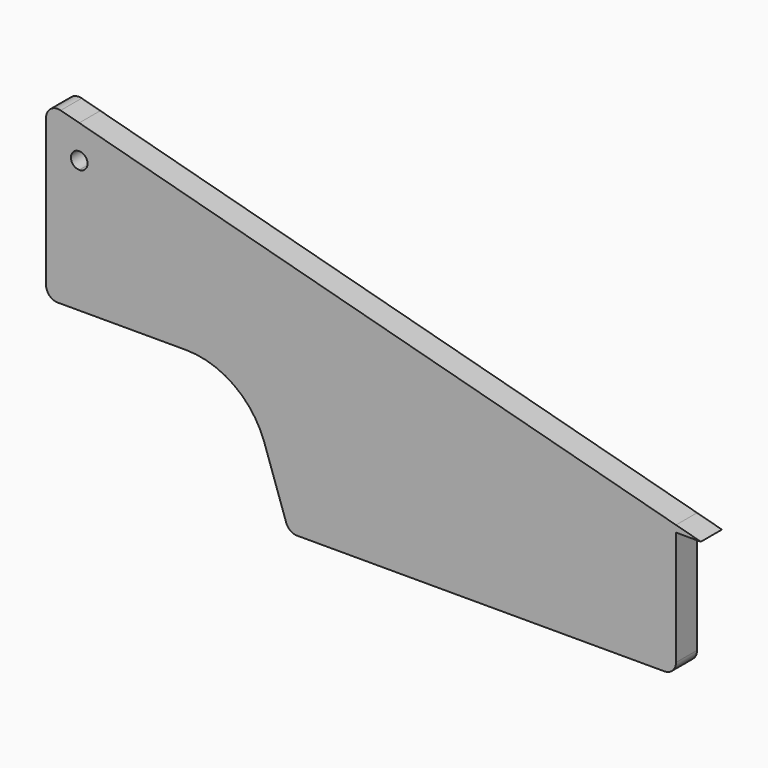
from build123d import *

# Parameters (mm, degrees)
F1_DEPTH = 1.5875


# Not quite as in the source:
# - a length typed as a fraction of an inch, garbled in the dataset ("3 / 203.2 mm" for 3/8 in), is restored


with BuildPart() as f1:
    # F0 (on Front) → F1 (new body)
    with BuildSketch(Plane.XZ):
        with BuildLine():
            ThreePointArc((-0.162727133, 0.4717287226), (0.0926759109, 0.1300044324), (0.4990071217, 0))
            Line((0.4990071217, 0), (22.65, 0))
            ThreePointArc((22.65, 0), (23.1449747468, 0.2050252532), (23.35, 0.7))
            Line((23.35, 0.7), (23.35, 7.5980762114))
            Line((23.35, 7.5980762114), (23.35, 8))
            Line((23.35, 8), (-12.65, 17.6461709275))
            Line((-12.65, 17.6461709275), (-12.65, 16.1461709275))
            ThreePointArc((-12.65, 16.1461709275), (-12.2964466094, 15.9997243181), (-12.15, 15.6461709275))
            ThreePointArc((-12.15, 15.6461709275), (-12.2964466094, 15.2926175369), (-12.65, 15.1461709275))
            Line((-12.65, 15.1461709275), (-12.65, 7.6820693124))
            Line((-12.65, 7.6820693124), (-6.2143365838, 7.6820693124))
            ThreePointArc((-6.2143365838, 7.6820693124), (-3.311970792, 6.7534662239), (-1.4876633356, 4.3125784367))
            Line((-1.4876633356, 4.3125784367), (-0.162727133, 0.4717287226))
        make_face()
        with BuildLine():
            Line((-13.95, 7.6820693124), (-12.65, 7.6820693124))
            Line((-12.65, 7.6820693124), (-12.65, 15.1461709275))
            ThreePointArc((-12.65, 15.1461709275), (-13.15, 15.6461709275), (-12.65, 16.1461709275))
            Line((-12.65, 16.1461709275), (-12.65, 17.6461709275))
            Line((-12.65, 17.6461709275), (-13.7688266684, 17.9459596298))
            ThreePointArc((-13.7688266684, 17.9459596298), (-14.3761330003, 17.8251588896), (-14.65, 17.2698115514))
            Line((-14.65, 17.2698115514), (-14.65, 8.3820693124))
            ThreePointArc((-14.65, 8.3820693124), (-14.4449747468, 7.8870945656), (-13.95, 7.6820693124))
        make_face()
        Polygon((23.35, 8), (23.35, 7.5980762114), (24.85, 7.5980762114), align=None)
    extrude(amount=F1_DEPTH)


solid = f1.part
